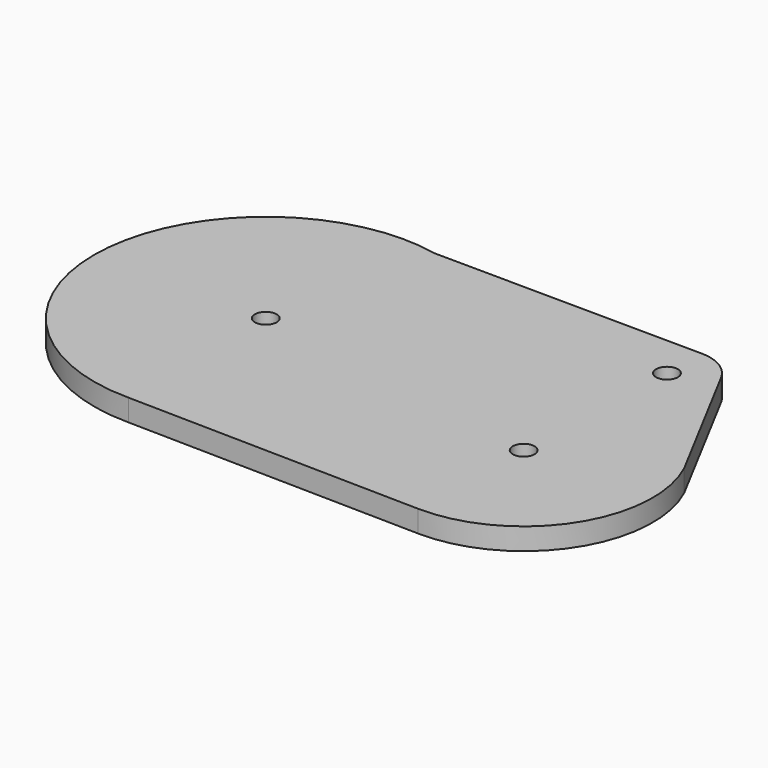
from build123d import *

# Parameters (mm, degrees)
F0_R     = 1.27
F1_DEPTH = 2.54


# Not quite as in the source:
# - a feature names something its author has since deleted; it is built from what else it names


with BuildPart() as f1:
    # F0 (on Top) → F1 (new body)
    with BuildSketch(Plane.XY):
        with BuildLine():
            Line((0, 14.3227163851), (-31.1715259044, 14.5573735897))
            ThreePointArc((-31.1715259044, 14.5573735897), (-55.1344730062, -2.9800210938), (-35.2392547778, -25.0245972461))
            Line((-35.2392547778, -25.0245972461), (-0.9759091536, -25.6627351613))
            ThreePointArc((-0.9759091536, -25.6627351613), (11.8962192038, -18.8265973986), (12.900298337, -4.2864360152))
            Line((12.900298337, -4.2864360152), (4.3965081654, 11.7041986386))
            ThreePointArc((4.3965081654, 11.7041986386), (2.5640325727, 13.627601953), (0, 14.3227163851))
        make_face()
        with Locations((-0.696967661, -10.6652775001)):
            Circle(F0_R, mode=Mode.SUBTRACT)
        with Locations((-35.2392547778, -5.0245972461)):
            Circle(F0_R, mode=Mode.SUBTRACT)
        with Locations((0, 9.3225747127)):
            Circle(F0_R, mode=Mode.SUBTRACT)
    extrude(amount=F1_DEPTH)


solid = f1.part
